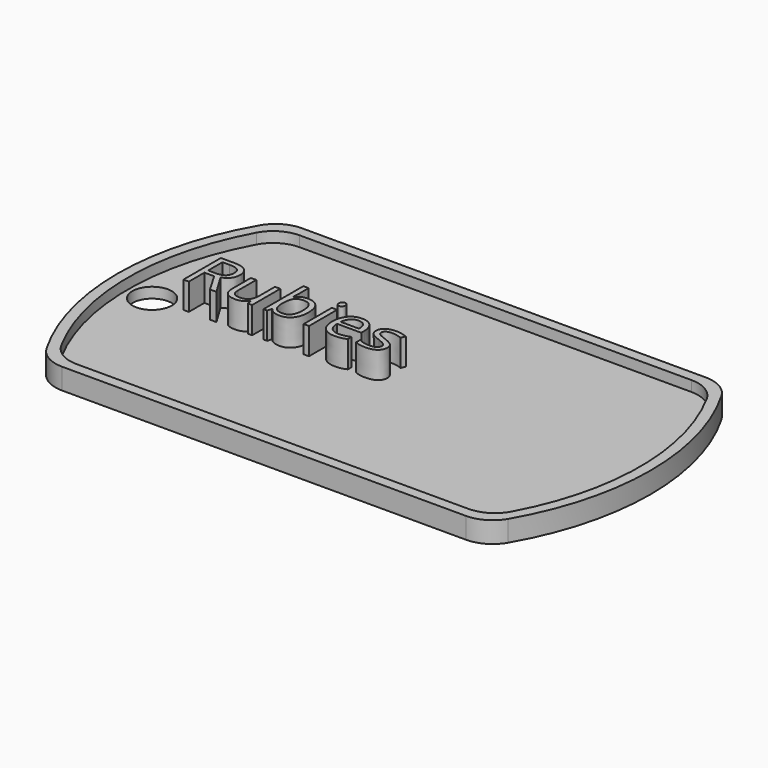
from build123d import *

# Parameters (mm, degrees)
F0_R         = 1.8739594118
F1_DEPTH     = 1
F3_DEPTH     = 1
F4_TEXT_SIZE = 6.254667662
F5_DEPTH     = 2.54


# Not quite as in the source:
# - Text() gives the source's letters only with a copy of the font that has no kerning and outlines rounded to 1/6400 em; it was checked with that copy


with BuildPart() as f1:
    # F0 (on Top) → F1 (new body)
    with BuildSketch(Plane.XY):
        with BuildLine():
            ThreePointArc((-19.2474145991, 14.2875), (-20.8349145991, 13.862130657), (-21.9970452561, 12.7))
            ThreePointArc((-21.9970452561, 12.7), (-25.4, 0), (-21.9970452561, -12.7))
            ThreePointArc((-21.9970452561, -12.7), (-20.8349145991, -13.862130657), (-19.2474145991, -14.2875))
            Line((-19.2474145991, -14.2875), (19.2474145991, -14.2875))
            ThreePointArc((19.2474145991, -14.2875), (20.8349145991, -13.862130657), (21.9970452561, -12.7))
            ThreePointArc((21.9970452561, -12.7), (25.4, 0), (21.9970452561, 12.7))
            ThreePointArc((21.9970452561, 12.7), (20.8349145991, 13.862130657), (19.2474145991, 14.2875))
            Line((19.2474145991, 14.2875), (-19.2474145991, 14.2875))
        make_face()
        with Locations((-22.0978986472, 0)):
            Circle(F0_R, mode=Mode.SUBTRACT)
    extrude(amount=F1_DEPTH)

    # F2 (on face) → F3 (join)
    with BuildSketch(Plane.XY.offset(1)):
        with BuildLine():
            Line((19.2474145991, 14.2875), (-19.2474145991, 14.2875))
            ThreePointArc((-19.2474145991, 14.2875), (-20.8349145991, 13.862130657), (-21.9970452561, 12.7))
            ThreePointArc((-21.9970452561, 12.7), (-25.4, 0), (-21.9970452561, -12.7))
            ThreePointArc((-21.9970452561, -12.7), (-20.8349145991, -13.862130657), (-19.2474145991, -14.2875))
            Line((-19.2474145991, -14.2875), (19.2474145991, -14.2875))
            ThreePointArc((19.2474145991, -14.2875), (20.8349145991, -13.862130657), (21.9970452561, -12.7))
            ThreePointArc((21.9970452561, -12.7), (25.4, 0), (21.9970452561, 12.7))
            ThreePointArc((21.9970452561, 12.7), (20.8349145991, 13.862130657), (19.2474145991, 14.2875))
        make_face()
        with BuildLine():
            ThreePointArc((-21.4526124879, 11.6252061249), (-20.2856017842, 12.8404540819), (-18.6611352482, 13.2875))
            Line((-18.6611352482, 13.2875), (18.6611352482, 13.2875))
            ThreePointArc((18.6611352482, 13.2875), (20.2856017842, 12.8404540819), (21.4526124879, 11.6252061249))
            ThreePointArc((21.4526124879, 11.6252061249), (24.4, 0), (21.4526124879, -11.6252061249))
            ThreePointArc((21.4526124879, -11.6252061249), (20.2856017842, -12.8404540819), (18.6611352482, -13.2875))
            Line((18.6611352482, -13.2875), (-18.6611352482, -13.2875))
            ThreePointArc((-18.6611352482, -13.2875), (-20.2856017842, -12.8404540819), (-21.4526124879, -11.6252061249))
            ThreePointArc((-21.4526124879, -11.6252061249), (-24.4, 0), (-21.4526124879, 11.6252061249))
        make_face(mode=Mode.SUBTRACT)
    extrude(amount=F3_DEPTH)

    # F4 (on face) → F5 (join)
    with BuildSketch(Plane.XY.offset(1)):
        with Locations((-19.7315218899, 0)):
            Text('Rubies', F4_TEXT_SIZE, font='Open Sans', text_align=(TextAlign.LEFT, TextAlign.BOTTOM))
    extrude(amount=F5_DEPTH)


solid = f1.part
